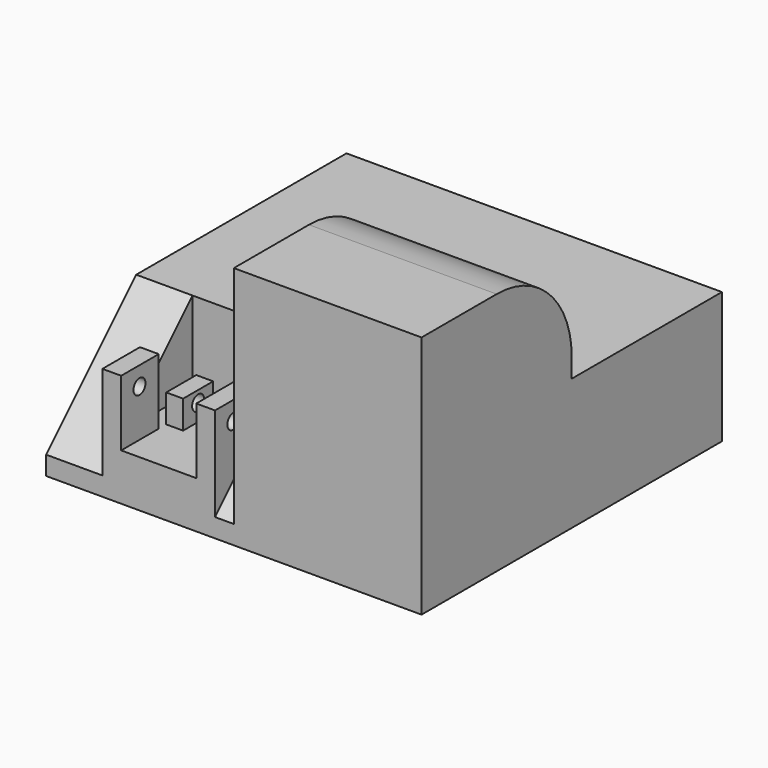
from build123d import *

# Parameters (mm, degrees)
F1_DEPTH  = 70
F0_W      = 100
F0_H      = 100
F2_DEPTH  = 130
F3_R      = 50
F4_SIZE   = 60
F0_W_2    = 10
F0_H_2    = 25
F5_DEPTH  = 60
F0_W_3    = 9
F0_H_3    = 20
F6_DEPTH  = 25
F7_DEPTH  = 40
F9_R      = 4
F10_DEPTH = 21
F11_DEPTH = 36.4


with BuildPart() as f1:
    # F0 (on Top) → F1 (new body)
    with BuildSketch(Plane.XY):
        Polygon((-10, -100), (0, -100), (0, 0), (100, 0), (100, 100), (-100, 100), (-100, -100), (-80, -100), (-70, -100), (-70, -75), (-70, -40), (-10, -40), (-10, -75), align=None)
    extrude(amount=F1_DEPTH)

    # F0 (on Top) → F2 (join)
    with BuildSketch(Plane.XY):
        with Locations((50, -50)):
            Rectangle(F0_W, F0_H)
    extrude(amount=F2_DEPTH)

    # F3
    f3_edges = [f1.edges().sort_by_distance(p)[0] for p in [
        (50, 0, 130),
    ]]
    fillet(f3_edges, radius=F3_R)

    # F4
    f4_edges = [f1.edges().sort_by_distance(p)[0] for p in [
        (-85, -100, 70),
        (-5, -100, 70),
    ]]
    chamfer(f4_edges, length=F4_SIZE)

    # F0 (on Top) → F5 (join)
    with BuildSketch(Plane.XY):
        with Locations((-65, -87.5)):
            Rectangle(F0_W_2, F0_H_2)
        with Locations((-15, -87.5)):
            Rectangle(F0_W_2, F0_H_2)
    extrude(amount=F5_DEPTH)

    # F0 (on Top) → F6 (join)
    with BuildSketch(Plane.XY):
        Polygon((-60, -100), (-20, -100), (-20, -75), (-10, -75), (-10, -40), (-70, -40), (-70, -75), (-60, -75), align=None)
        with Locations((-55.5, -60)):
            Rectangle(F0_W_3, F0_H_3, mode=Mode.SUBTRACT)
        with Locations((-24.5, -60)):
            Rectangle(F0_W_3, F0_H_3, mode=Mode.SUBTRACT)
    extrude(amount=F6_DEPTH)

    # F0 (on Top) → F7 (join)
    with BuildSketch(Plane.XY):
        with Locations((-24.5, -60)):
            Rectangle(F0_W_3, F0_H_3)
        with Locations((-55.5, -60)):
            Rectangle(F0_W_3, F0_H_3)
    extrude(amount=F7_DEPTH)

    # F9 (on offset) → F10 (cut, symmetric)
    with BuildSketch(Plane.YZ.offset(-45)):
        with Locations((-60, 34)):
            Circle(F9_R)
    extrude(amount=F10_DEPTH, both=True, mode=Mode.SUBTRACT)

    # F9 (on offset) → F11 (cut, symmetric)
    with BuildSketch(Plane.YZ.offset(-45)):
        with Locations((-87.799012661, 50)):
            Circle(F9_R)
    extrude(amount=F11_DEPTH, both=True, mode=Mode.SUBTRACT)


solid = f1.part
